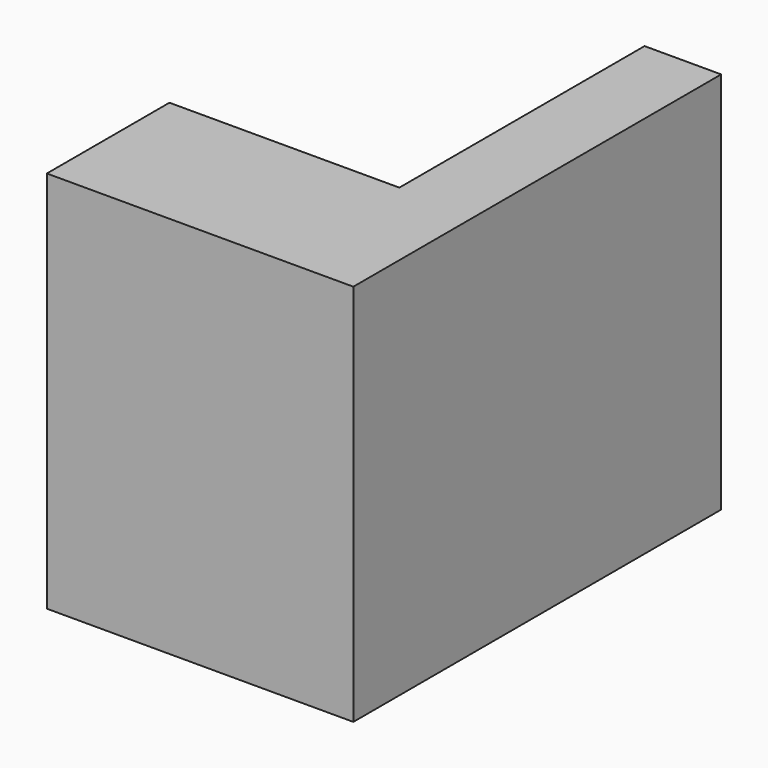
from build123d import *

# Parameters (mm, degrees)
F0_W     = 25.4
F0_H     = 31.75
F1_DEPTH = 38.1
F3_DEPTH = 25.4


# Not quite as in the source:
# - a length typed as a fraction of an inch, garbled in the dataset ("3 / 203.2 mm" for 3/8 in), is restored


with BuildPart() as f1:
    # F0 (on Front) → F1 (new body)
    with BuildSketch(Plane.XZ):
        with Locations((9.313e-07, 20.9670082225)):
            Rectangle(F0_W, F0_H)
    extrude(amount=F1_DEPTH)

    # F2 (on Front) → F3 (cut)
    with BuildSketch(Plane.XZ):
        Polygon((-12.6999990687, 11.4420082225), (6.3500009313, 36.8420082225), (-12.6999990687, 36.8420082225), align=None)
    extrude(amount=F3_DEPTH, mode=Mode.SUBTRACT)


solid = f1.part
